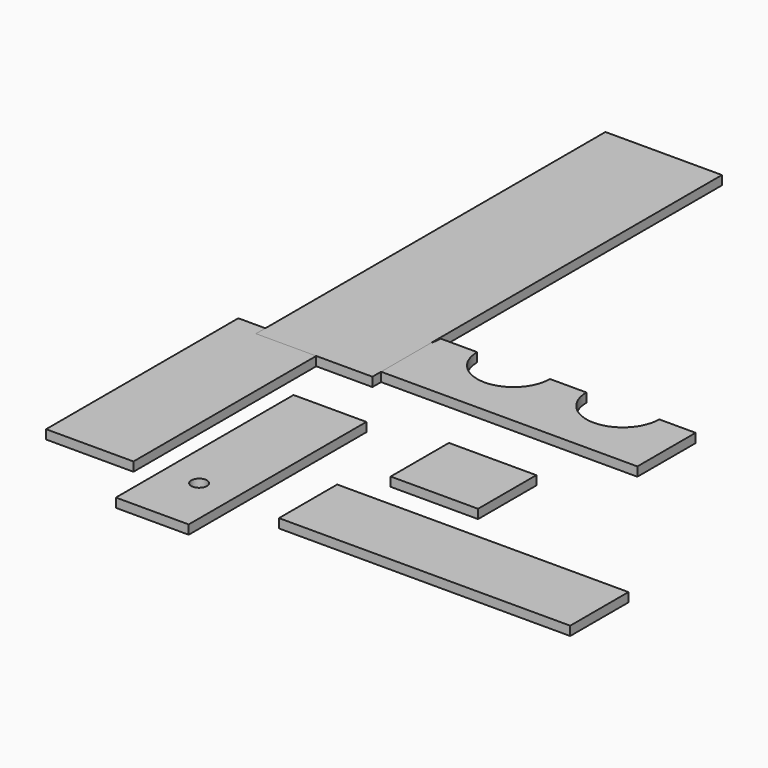
from build123d import *

# Parameters (mm, degrees)
F1_DEPTH  = 3.175
F2_W      = 30.48
F2_H      = 83.82
F3_DEPTH  = 3.175
F4_W      = 25.4
F4_H      = 77.47
F4_R      = 2.7154298689
F5_DEPTH  = 3.175
F6_W      = 30.48
F6_H      = 25.4
F7_DEPTH  = 3.175
F8_W      = 101.6
F8_H      = 25.4
F9_DEPTH  = 3.175
F10_W     = 40.64
F10_H     = 152.4
F11_DEPTH = 3.175


# Not quite as in the source:
# - a length typed as a fraction of an inch, garbled in the dataset ("3 / 203.2 mm" for 3/8 in), is restored


with BuildPart() as f1:
    # F0 (on Top) → F1 (new body)
    with BuildSketch(Plane.XY):
        with BuildLine():
            Line((-52.0695035428, 39.5263851967), (-64.7695035428, 39.5263851967))
            Line((-64.7695035428, 39.5263851967), (-64.7695035428, 14.1263851967))
            Line((-64.7695035428, 14.1263851967), (62.2304964572, 14.1263851967))
            Line((62.2304964572, 14.1263851967), (62.2304964572, 39.5263851967))
            Line((62.2304964572, 39.5263851967), (49.5304964572, 39.5263851967))
            ThreePointArc((49.5304964572, 39.5263851967), (36.8304964572, 26.8263851967), (24.1304964572, 39.5263851967))
            Line((24.1304964572, 39.5263851967), (11.4304964572, 39.5263851967))
            ThreePointArc((11.4304964572, 39.5263851967), (-1.2695035428, 26.8263851967), (-13.9695035428, 39.5263851967))
            Line((-13.9695035428, 39.5263851967), (-26.6695035428, 39.5263851967))
            ThreePointArc((-26.6695035428, 39.5263851967), (-39.3695035428, 26.8263851967), (-52.0695035428, 39.5263851967))
        make_face()
    extrude(amount=F1_DEPTH)


with BuildPart() as f3:
    # F2 (on Top) → F3 (new body)
    with BuildSketch(Plane.XY):
        with Locations((-62.027904564, -27.4314320334)):
            Rectangle(F2_W, F2_H)
    extrude(amount=F3_DEPTH)


with BuildPart() as f5:
    # F4 (on Top) → F5 (new body)
    with BuildSketch(Plane.XY):
        with Locations((-24.5303590782, -50.2138879341)):
            Rectangle(F4_W, F4_H)
        with Locations((-24.811277166, -68.1698620319)):
            Circle(F4_R, mode=Mode.SUBTRACT)
    extrude(amount=F5_DEPTH)


with BuildPart() as f7:
    # F6 (on Top) → F7 (new body)
    with BuildSketch(Plane.XY):
        with Locations((28.7132419021, -19.8017735619)):
            Rectangle(F6_W, F6_H)
    extrude(amount=F7_DEPTH)


with BuildPart() as f9:
    # F8 (on Top) → F9 (new body)
    with BuildSketch(Plane.XY):
        with Locations((55.8379401919, -57.9767658847)):
            Rectangle(F8_W, F8_H)
    extrude(amount=F9_DEPTH)


with BuildPart() as f11:
    # F10 (on Top) → F11 (new body)
    with BuildSketch(Plane.XY):
        with Locations((-47.5000926219, 86.5590404719)):
            Rectangle(F10_W, F10_H)
    extrude(amount=F11_DEPTH)


solid = Compound([f1.part, f3.part, f5.part, f7.part, f9.part, f11.part])
